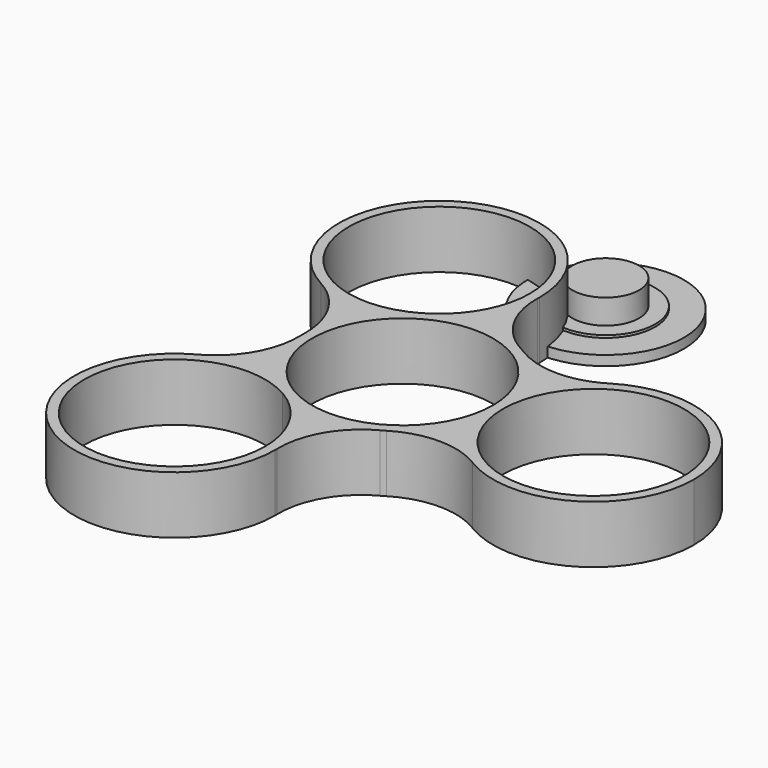
from build123d import *

# Parameters (mm, degrees)
F1_DEPTH = 7
F2_R     = 10
F3_R     = 9.5
F4_DEPTH = 1.2
F5_R     = 6
F6_DEPTH = 0.3
F7_R     = 4.05
F8_DEPTH = 3


with BuildPart() as f1:
    # F0 (on Top) → F1 (new body)
    with BuildSketch(Plane.XY):
        with BuildLine():
            ThreePointArc((0.6, 20.0917893678), (-21.0782412309, 27.7731266973), (-9.0726136344, 8.1564503211))
            ThreePointArc((-9.0726136344, 8.1564503211), (-7.6813368071, 9.4782416543), (-6.0999988352, 10.5655105986))
            ThreePointArc((-6.0999988352, 10.5655105986), (-4.3677283965, 11.3913541186), (-2.5273863656, 11.9353390467))
            ThreePointArc((-2.5273863656, 11.9353390467), (-0.2086461222, 15.7240603434), (0.6, 20.0917893678))
        make_face()
        with BuildLine():
            ThreePointArc((-0.6, 20.0917893678), (-2.0737202221, 14.5917899502), (-6.0999988352, 10.5655105986))
            ThreePointArc((-6.0999988352, 10.5655105986), (-21.1262797779, 25.5917887854), (-0.6, 20.0917893678))
        make_face(mode=Mode.SUBTRACT)
        with BuildLine():
            ThreePointArc((-5.500001168, 9.5262787673), (5.499999416, 9.5262797788), (11, 0))
            ThreePointArc((11, 0), (11.1509336461, 1.913112647), (11.6, 3.7788887255))
            ThreePointArc((11.6, 3.7788887255), (6.1, 10.5655099262), (-2.5273863656, 11.9353390467))
            ThreePointArc((-2.5273863656, 11.9353390467), (-3.9186631944, 10.6135477124), (-5.500001168, 9.5262787673))
        make_face()
        with BuildLine():
            ThreePointArc((-9.0726136344, 8.1564503211), (-7.2322716053, 8.7004352486), (-5.500001168, 9.5262787673))
            ThreePointArc((-5.500001168, 9.5262787673), (-3.9186631944, 10.6135477124), (-2.5273863656, 11.9353390467))
            ThreePointArc((-2.5273863656, 11.9353390467), (-4.3677283965, 11.3913541186), (-6.0999988352, 10.5655105986))
            ThreePointArc((-6.0999988352, 10.5655105986), (-7.6813368071, 9.4782416543), (-9.0726136344, 8.1564503211))
        make_face()
        with BuildLine():
            ThreePointArc((11.6, -3.7788887255), (11.1509336461, -1.913112647), (11, 0))
            ThreePointArc((11, 0), (5.4999994158, -9.5262797789), (-5.5000011684, -9.526278767))
            ThreePointArc((-5.5000011684, -9.526278767), (-3.9186631946, -10.6135477122), (-2.5273863656, -11.9353390467))
            ThreePointArc((-2.5273863656, -11.9353390467), (6.1, -10.5655099262), (11.6, -3.7788887255))
        make_face()
        with BuildLine():
            ThreePointArc((11.6, 3.7788887255), (11.1509336461, 1.913112647), (11, 0))
            ThreePointArc((11, 0), (11.1509336461, -1.913112647), (11.6, -3.7788887255))
            ThreePointArc((11.6, -3.7788887255), (12.0490663539, -1.913112647), (12.2, 0))
            ThreePointArc((12.2, 0), (12.0490663539, 1.913112647), (11.6, 3.7788887255))
        make_face()
        with BuildLine():
            ThreePointArc((35.4, 0), (25.113112647, 12.0490663539), (11.6, 3.7788887255))
            ThreePointArc((11.6, 3.7788887255), (12.0490663539, 1.913112647), (12.2, 0))
            ThreePointArc((12.2, 0), (12.0490663539, -1.913112647), (11.6, -3.7788887255))
            ThreePointArc((11.6, -3.7788887255), (25.113112647, -12.0490663539), (35.4, 0))
        make_face()
        with BuildLine():
            ThreePointArc((34.2, 0), (23.2, -11), (12.2, 0))
            ThreePointArc((12.2, 0), (23.2, 11), (34.2, 0))
        make_face(mode=Mode.SUBTRACT)
        with BuildLine():
            ThreePointArc((-5.5000011684, -9.526278767), (-11, 3e-10), (-5.500001168, 9.5262787673))
            ThreePointArc((-5.500001168, 9.5262787673), (-7.2322716053, 8.7004352486), (-9.0726136344, 8.1564503211))
            ThreePointArc((-9.0726136344, 8.1564503211), (-12.2, 0), (-9.0726136344, -8.1564503211))
            ThreePointArc((-9.0726136344, -8.1564503211), (-7.2322716055, -8.7004352485), (-5.5000011684, -9.526278767))
        make_face()
        with BuildLine():
            ThreePointArc((-2.5273863656, -11.9353390467), (-3.9186631946, -10.6135477122), (-5.5000011684, -9.526278767))
            ThreePointArc((-5.5000011684, -9.526278767), (-7.2322716055, -8.7004352485), (-9.0726136344, -8.1564503211))
            ThreePointArc((-9.0726136344, -8.1564503211), (-7.6813368071, -9.4782416543), (-6.0999988352, -10.5655105986))
            ThreePointArc((-6.0999988352, -10.5655105986), (-4.3677283965, -11.3913541186), (-2.5273863656, -11.9353390467))
        make_face()
        with BuildLine():
            ThreePointArc((0.6, -20.0917893678), (-0.2086461222, -15.7240603434), (-2.5273863656, -11.9353390467))
            ThreePointArc((-2.5273863656, -11.9353390467), (-4.3677283965, -11.3913541186), (-6.0999988352, -10.5655105986))
            ThreePointArc((-6.0999988352, -10.5655105986), (-7.6813368071, -9.4782416543), (-9.0726136344, -8.1564503211))
            ThreePointArc((-9.0726136344, -8.1564503211), (-21.0782412309, -27.7731266973), (0.6, -20.0917893678))
        make_face()
        with BuildLine():
            ThreePointArc((-0.6, -20.0917893678), (-21.1262797779, -25.5917887854), (-6.0999988352, -10.5655105986))
            ThreePointArc((-6.0999988352, -10.5655105986), (-2.0737202221, -14.5917899502), (-0.6, -20.0917893678))
        make_face(mode=Mode.SUBTRACT)
    extrude(amount=F1_DEPTH)

    # F2
    f2_edges = [f1.edges().sort_by_distance(p)[0] for p in [
        (-9.072614, 8.15645, 3.5),
        (11.6, -3.778889, 3.5),
        (11.6, 3.778889, 3.5),
        (-2.527386, 11.935339, 3.5),
        (-2.527386, -11.935339, 3.5),
        (-9.072614, -8.15645, 3.5),
    ]]
    fillet(f2_edges, radius=F2_R)


with BuildPart() as f4:
    # F3 (on Top) → F4 (new body)
    with BuildSketch(Plane.XY):
        with Locations((0, 30.8597814292)):
            Circle(F3_R)
    extrude(amount=F4_DEPTH)

    # F5 (on face) → F6 (join)
    with BuildSketch(Plane.XY.offset(1.2)):
        with Locations((0, 30.8597814292)):
            Circle(F5_R)
    extrude(amount=F6_DEPTH)

    # F7 (on face) → F8 (join)
    with BuildSketch(Plane.XY.offset(1.5)):
        with Locations((0, 30.8597814292)):
            Circle(F7_R)
    extrude(amount=F8_DEPTH)

    # F9 (on Right) → F10 (revolve, cut)
    with BuildSketch(Plane.YZ):
        with BuildLine():
            ThreePointArc((30.8597814292, 0.6), (26.499448873, 0.4498220638), (22.1597814292, 0))
            Line((22.1597814292, 0), (30.8597814292, 0))
            Line((30.8597814292, 0), (30.8597814292, 0.6))
        make_face()
    revolve(axis=Axis((0, 30.8597814292, 0.3), (0, 0, -1)), mode=Mode.SUBTRACT)


solid = Compound([f1.part, f4.part])
